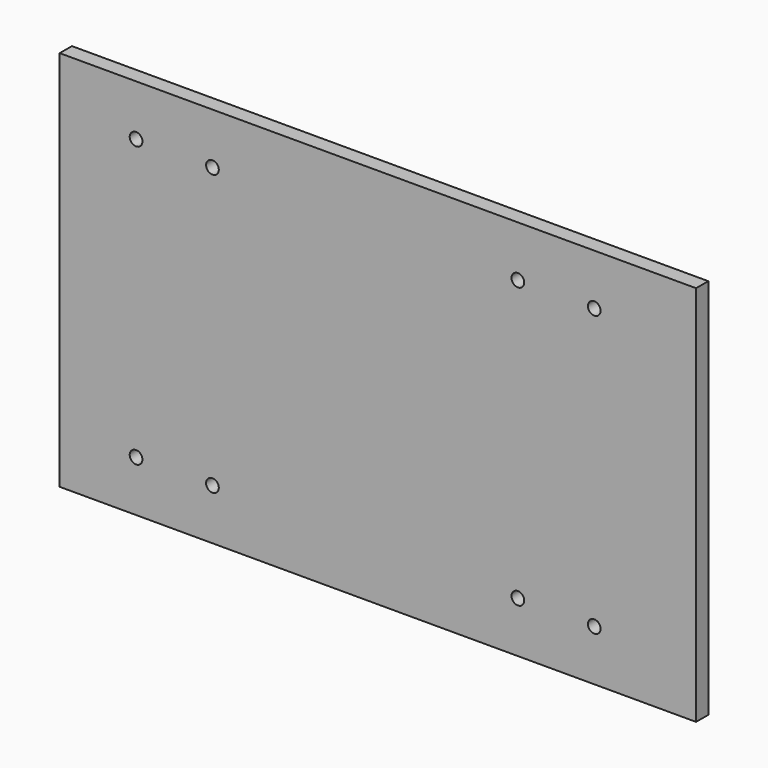
from build123d import *

# Parameters (mm, degrees)
F0_W     = 250
F0_H     = 150
F0_R     = 2.5
F1_DEPTH = 6


# Not quite as in the source:
# - a feature names something its author has since deleted; it is built from what else it names


with BuildPart() as f1:
    # F0 (on Front) → F1 (new body)
    with BuildSketch(Plane.XZ):
        Rectangle(F0_W, F0_H)
        with Locations((-95, -55)):
            Circle(F0_R, mode=Mode.SUBTRACT)
        with Locations((-65, -55)):
            Circle(F0_R, mode=Mode.SUBTRACT)
        with Locations((55, -55)):
            Circle(F0_R, mode=Mode.SUBTRACT)
        with Locations((85, -55)):
            Circle(F0_R, mode=Mode.SUBTRACT)
        with Locations((-95, 55)):
            Circle(F0_R, mode=Mode.SUBTRACT)
        with Locations((-65, 55)):
            Circle(F0_R, mode=Mode.SUBTRACT)
        with Locations((55, 55)):
            Circle(F0_R, mode=Mode.SUBTRACT)
        with Locations((85, 55)):
            Circle(F0_R, mode=Mode.SUBTRACT)
    extrude(amount=F1_DEPTH)


solid = f1.part
